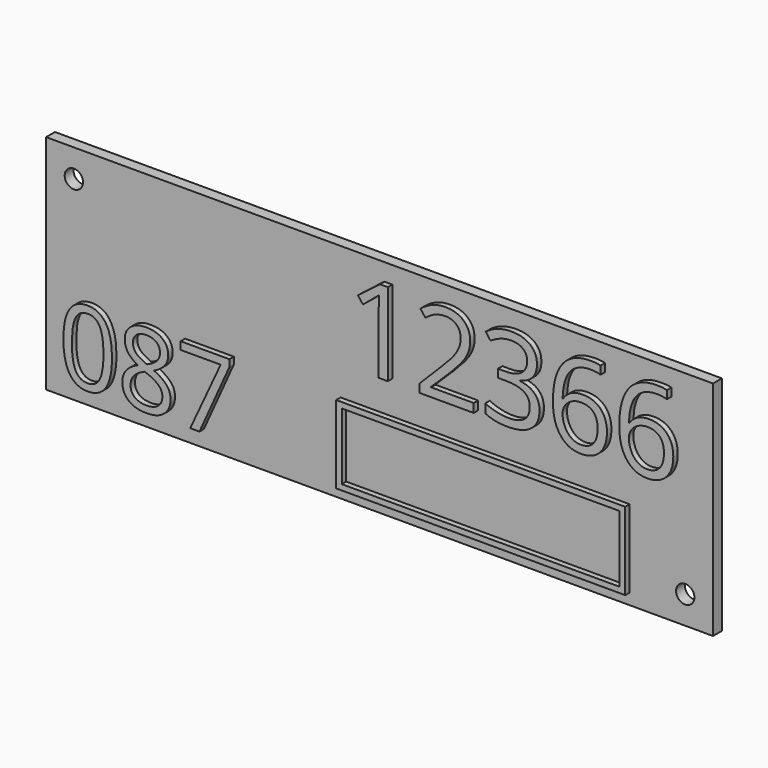
from build123d import *

# Parameters (mm, degrees)
F0_W         = 120
F0_H         = 40
F1_DEPTH     = 2
F3_D         = 3.3
F4_TEXT_SIZE = 20.871833895
F5_DEPTH     = 1
F6_TEXT_SIZE = 18.5054667028
F7_DEPTH     = 1
F8_W         = 52
F8_H         = 14
F8_W_2       = 49.99999962
F8_H_2       = 11.99999962
F9_DEPTH     = 1


# Not quite as in the source:
# - Text() gives the source's letters only with a copy of the font that has no kerning and outlines rounded to 1/6400 em; it was checked with that copy


with BuildPart() as f1:
    # F0 (on Front) → F1 (new body)
    with BuildSketch(Plane.XZ):
        Rectangle(F0_W, F0_H)
    extrude(amount=F1_DEPTH)

    # F3 (through all)
    with Locations(Plane.XZ.offset(2)):
        with Locations((-55, 15), (55, -15)):
            Hole(F3_D / 2)

    # F4 (on face) → F5 (join)
    with BuildSketch(Plane.XZ.offset(2)):
        with Locations((-5, 2)):
            Text('12366', F4_TEXT_SIZE, font='Open Sans', text_align=(TextAlign.LEFT, TextAlign.BOTTOM))
    extrude(amount=F5_DEPTH)

    # F6 (on face) → F7 (join)
    with BuildSketch(Plane.XZ.offset(2)):
        with Locations((-57, -17)):
            Text('087', F6_TEXT_SIZE, font='Open Sans', text_align=(TextAlign.LEFT, TextAlign.BOTTOM))
    extrude(amount=F7_DEPTH)

    # F8 (on face) → F9 (join)
    with BuildSketch(Plane.XZ.offset(2)):
        with Locations((19, -11)):
            Rectangle(F8_W, F8_H)
        with Locations((19, -11)):
            Rectangle(F8_W_2, F8_H_2, mode=Mode.SUBTRACT)
    extrude(amount=F9_DEPTH)


solid = f1.part
